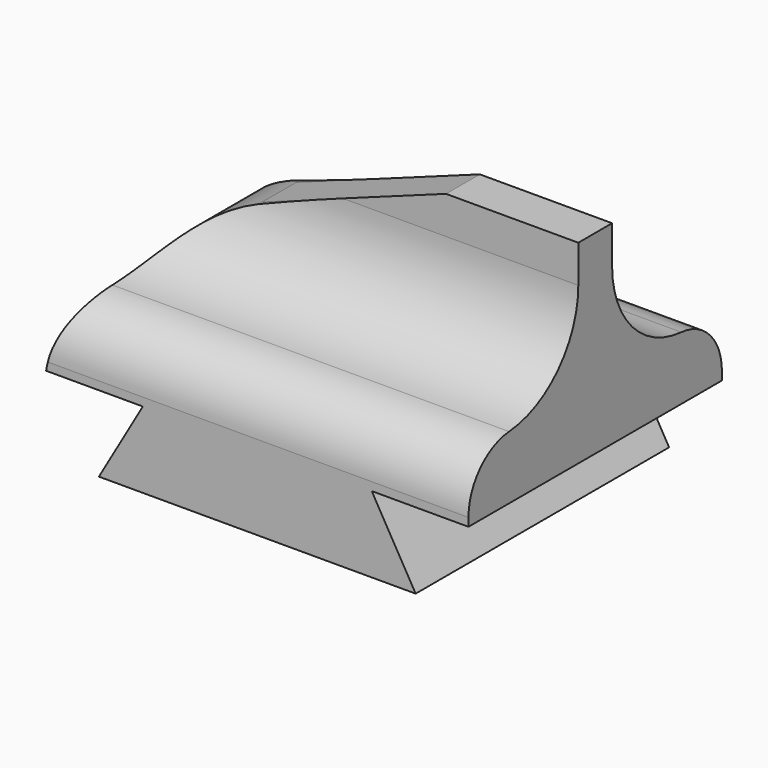
from build123d import *

# Parameters (mm, degrees)
F0_W         = 9.525
F0_H         = 9.525
F1_DEPTH     = 2.286
F2_T1_DEPTH  = 21.3619144247
F3_W         = 2.9083
F3_H         = 9.525
F3_W_2       = 6.8834
F4_DEPTH     = 1.905
F5_R         = 1.6556676611
F6_W         = 12.7
F6_H         = 1.27
F7_DEPTH     = 3.937
F8_SIZE2     = 8.7232408068
F8_SIZE      = 3.175
F9_T4_DEPTH  = 12.7
F9_T9_DEPTH  = 12.7
F10_T1_DEPTH = 20.3689561099


# Not quite as in the source:
# - a fillet or chamfer that OpenCascade refuses, or shapes differently, is made with other operations: its cross-section is extruded or revolved along the edge and cut away or added


with BuildPart() as f1:
    # F0 (on Top) → F1 (new body)
    with BuildSketch(Plane.XY):
        Rectangle(F0_W, F0_H)
    extrude(amount=F1_DEPTH)

    # F2: chamfer of 1.3208 x 2.2876927066 on 2 edges, made by hand

    # F2_s2 → F2_t1 (cut)
    with BuildSketch(Plane.XZ.offset(-10.6809572123)):
        Polygon((-4.7625, -0.0016927066), (-3.4417, 2.286), (-4.7625, 2.286), align=None)
        Polygon((4.7625, -0.0016927066), (3.4417, 2.286), (4.7625, 2.286), align=None)
    extrude(amount=F2_T1_DEPTH, mode=Mode.SUBTRACT)

    # F3 (on face) → F4 (join)
    with BuildSketch(Plane.XY.offset(2.286)):
        with Locations((4.89585, 0)):
            Rectangle(F3_W, F3_H)
        Rectangle(F3_W_2, F3_H)
        with Locations((-4.89585, 0)):
            Rectangle(F3_W, F3_H)
    extrude(amount=F4_DEPTH)

    # F5
    f5_edges = [f1.edges().sort_by_distance(p)[0] for p in [
        (0, 4.7625, 4.191),
        (0, -4.7625, 4.191),
    ]]
    fillet(f5_edges, radius=F5_R)

    # F6 (on face) → F7 (join)
    with BuildSketch(Plane.XY.offset(4.191)):
        Rectangle(F6_W, F6_H)
    extrude(amount=F7_DEPTH)

    # F8
    f8_edges = [f1.edges().sort_by_distance(p)[0] for p in [
        (-6.35, 0, 8.128),
    ]]
    f8_side = f1.faces().sort_by_distance((-6.35, 0, 3.872106))[0]
    chamfer(f8_edges, length=F8_SIZE, length2=F8_SIZE2, reference=f8_side)

    # F9: fillet of radius 2.8207671263 on 2 edges, made by hand


with BuildPart() as f9_tool2:
    # F9_s3 → F9_t4 (new body)
    with BuildSketch(Plane.YZ.offset(-6.35)):
        with BuildLine():
            ThreePointArc((-0.635, 6.9981468006), (-1.3849039981, 5.0828783899), (-3.235890411, 4.1859623453))
            Line((-3.235890411, 4.1859623453), (-3.2139027394, 3.9047438998))
            ThreePointArc((-3.2139027394, 3.9047438998), (-3.1068323389, 3.9089232874), (-0.635, 3.9089232874))
            Line((-0.635, 3.9089232874), (-0.3529232874, 4.191))
            Line((-0.3529232874, 4.191), (-0.3529232874, 6.9981468006))
            Line((-0.3529232874, 6.9981468006), (-0.635, 6.9981468006))
        make_face()
    extrude(amount=F9_T4_DEPTH)

    split(bisect_by=Plane(origin=(-2.3346724085, 0, 6.4144597241), x_dir=(0, 1, 0), z_dir=(0.3420201433, 0, -0.9396926208)), keep=Keep.TOP)


with BuildPart() as f1_1:
    add(f1.part)

    # F9_t1: union F9_tool2
    add(f9_tool2.part)


with BuildPart() as f9_tool7:
    # F9_s8 → F9_t9 (new body)
    with BuildSketch(Plane.YZ.offset(6.35)):
        with BuildLine():
            ThreePointArc((0.635, 6.9981468006), (1.3849039981, 5.0828783899), (3.235890411, 4.1859623453))
            Line((3.235890411, 4.1859623453), (3.2139027394, 3.9047438998))
            ThreePointArc((3.2139027394, 3.9047438998), (3.1068323389, 3.9089232874), (0.635, 3.9089232874))
            Line((0.635, 3.9089232874), (0.3529232874, 4.191))
            Line((0.3529232874, 4.191), (0.3529232874, 6.9981468006))
            Line((0.3529232874, 6.9981468006), (0.635, 6.9981468006))
        make_face()
    extrude(amount=-F9_T9_DEPTH)

    split(bisect_by=Plane(origin=(-2.3346724085, 0, 6.4144597241), x_dir=(0, 1, 0), z_dir=(0.3420201433, 0, -0.9396926208)), keep=Keep.TOP)


with BuildPart() as f1_2:
    add(f1_1.part)

    # F9_t6: union F9_tool7
    add(f9_tool7.part)

    # F10: fillet of radius 5.08 on 1 edges, made by hand

    # F10_s2 → F10_t1 (cut)
    with BuildSketch(Plane.XZ.offset(-10.184478055)):
        with BuildLine():
            ThreePointArc((-6.3503933611, 2.2860725742), (-5.2327762913, 4.646139378), (-3.0907506998, 6.1396954024))
            Line((-3.0907506998, 6.1396954024), (-3.2645725807, 6.6172670953))
            ThreePointArc((-3.2645725807, 6.6172670953), (-4.8941288268, 6.0237314555), (-6.5238218809, 5.4305716928))
            Line((-6.5238218809, 5.4305716928), (-6.8582211803, 4.953))
            ThreePointArc((-6.8582211803, 4.953), (-6.8582211803, 3.6195362871), (-6.8501795082, 2.3782819842))
            Line((-6.8501795082, 2.3782819842), (-6.3503933611, 2.2860725742))
        make_face()
    extrude(amount=F10_T1_DEPTH, mode=Mode.SUBTRACT)


solid = f1_2.part
